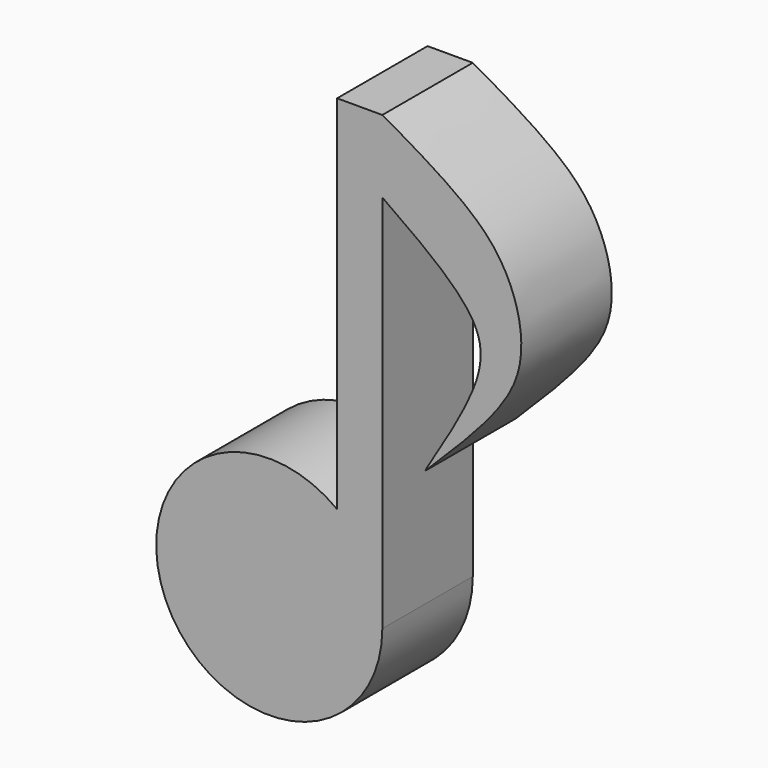
from build123d import *

# Parameters (mm, degrees)
F1_DEPTH = 10.16
F3_R     = 12.7
F4_DEPTH = 2.54
F5_DEPTH = 12.7
F6_W     = 6.4024168532
F6_H     = 4.7285845503
F7_DEPTH = 8.89


# Not quite as in the source:
# - a feature names something its author has since deleted; it is built from what else it names


with BuildPart() as f1:
    # F0 (on Front) → F1 (new body)
    with BuildSketch(Plane.XZ):
        with BuildLine():
            ThreePointArc((7.62, 10.16), (-11.3592253257, -5.6796126628), (12.7, 0))
            Line((12.7, 0), (10.16, 0))
            ThreePointArc((10.16, 0), (-9.5038097624, -3.5921024484), (7.62, 6.7202083301))
            Line((7.62, 6.7202083301), (7.62, 10.16))
        make_face()
        with BuildLine():
            Line((10.16, 0), (12.7, 0))
            ThreePointArc((12.7, 0), (11.3592253257, 5.6796126628), (7.62, 10.16))
            Line((7.62, 10.16), (7.62, 6.7202083301))
            ThreePointArc((7.62, 6.7202083301), (9.5038097624, 3.5921024484), (10.16, 0))
        make_face()
    extrude(amount=F1_DEPTH)

    # F3 (on offset) → F4 (join)
    with BuildSketch(Plane.XZ.offset(10.16)):
        Circle(F3_R)
    extrude(amount=F4_DEPTH)

    # F0 (on Front) → F5 (join)
    with BuildSketch(Plane.XZ):
        with BuildLine():
            ThreePointArc((7.62, 10.16), (11.3592253257, 5.6796126628), (12.7, 0))
            Line((12.7, 0), (12.7, 42.6425151527))
            Line((12.7, 42.6425151527), (12.7, 50.8))
            Line((12.7, 50.8), (7.62, 50.8))
            Line((7.62, 50.8), (7.62, 10.16))
        make_face()
        with BuildLine():
            Line((12.7, 50.8), (12.7, 42.6425151527))
            add(Edge.make_bspline(
                [(12.7, 42.6425151527), (16.4159388024, 40.0315705937), (22.9518647177, 35.4392075022), (24.9899073327, 28.3591527492), (17.7928973736, 17.9350558311), (17.5403915346, 17.1955488622)],
                knots=[0, 0, 0, 0, 0.3509731008, 0.6173229181, 0.9655230387, 0.9655230387, 0.9655230387, 0.9655230387], degree=3))
            add(Edge.make_bspline(
                [(17.5403915346, 17.1955488622), (21.2544211974, 20.8693964105), (27.3124893335, 26.8619222623), (28.6399816467, 32.8200369115), (27.7218714736, 37.874085965), (24.7037959914, 43.3162815788), (17.5887424866, 48.0374298627), (14.2146676642, 49.9440793479), (12.7, 50.8)],
                knots=[0, 0, 0, 0, 0.2328114889, 0.3797459877, 0.5165565754, 0.6708114391, 0.8522228182, 1, 1, 1, 1], degree=3))
        make_face()
    extrude(amount=F5_DEPTH)

    # F6 (on Front) → F7 (cut)
    with BuildSketch(Plane.XZ):
        with Locations((-0.0436579576, -11.8226897903)):
            Rectangle(F6_W, F6_H)
    extrude(amount=F7_DEPTH, mode=Mode.SUBTRACT)


solid = f1.part
